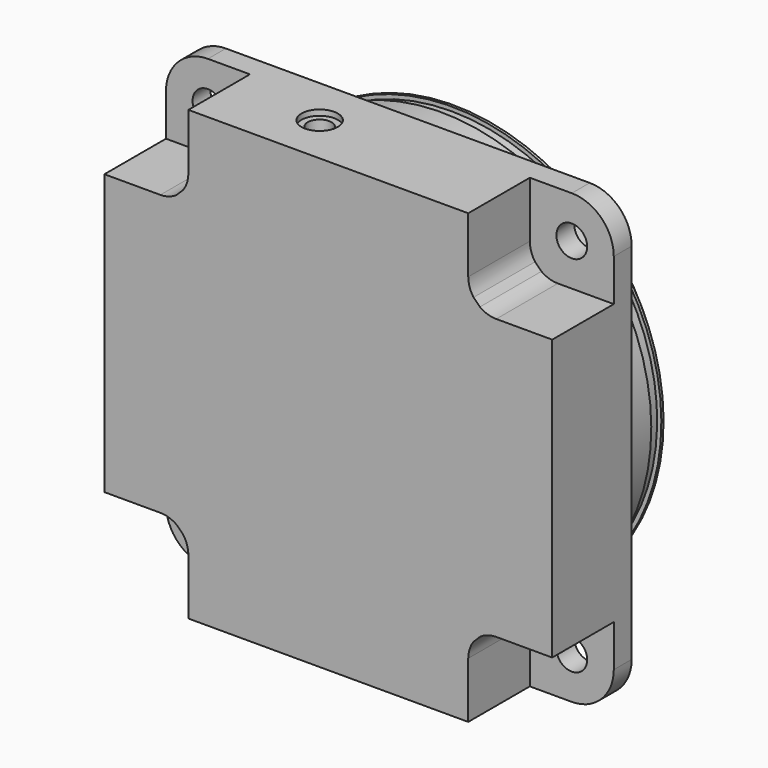
from build123d import *

# Parameters (mm, degrees)
F1_DEPTH        = 58
F0_R            = 5.5
F2_DEPTH        = 35.5
F3_DEPTH        = 35.5
F3_COPIES_COUNT = 4
F4_DEPTH        = 27.5
F4_COPIES_COUNT = 4
F5_SIZE         = 2
F7_D            = 8.5
F7_DEPTH        = 35
F7_CBORE_D      = 13
F7_CBORE_DEPTH  = 2
F7_TIP          = 2.5536576309
F9_D            = 8
F9_DEPTH        = 40
F9_TIP          = 2.4034424761
F10_W           = 4.5
F10_H           = 1.5


# Not quite as in the source:
# - a pattern or mirror of a feature is missing from the dataset's text; its kind, count and spacing are read off the source's solid


with BuildPart() as f1:
    # F0 (on Front) → F1 (new body)
    with BuildSketch(Plane.XZ):
        with BuildLine():
            ThreePointArc((-51.8845091547, 54.1571575119), (-52.9289321881, 52.9289321881), (-54.1571575119, 51.8845091547))
            ThreePointArc((-54.1571575119, 51.8845091547), (-27.9572279259, -69.5944926463), (75, 0))
            ThreePointArc((75, 0), (29.4419922338, 68.979483133), (-51.8845091547, 54.1571575119))
        make_face()
        with BuildLine():
            ThreePointArc((-51.8845091547, 54.1571575119), (-53.033008589, 53.033008589), (-54.1571575119, 51.8845091547))
            ThreePointArc((-54.1571575119, 51.8845091547), (-52.9289321881, 52.9289321881), (-51.8845091547, 54.1571575119))
        make_face()
    extrude(amount=-F1_DEPTH)

    # F0 (on Front) → F2 (join)
    with BuildSketch(Plane.XZ):
        with BuildLine():
            Line((-65, -80), (65, -80))
            ThreePointArc((65, -80), (75.6066017178, -75.6066017178), (80, -65))
            Line((80, -65), (80, 65))
            ThreePointArc((80, 65), (75.6066017178, 75.6066017178), (65, 80))
            Line((65, 80), (-50, 80))
            Line((-50, 80), (-50, 60))
            ThreePointArc((-50, 60), (-50.4827811717, 56.9303834484), (-51.8845091547, 54.1571575119))
            ThreePointArc((-51.8845091547, 54.1571575119), (29.4419922338, 68.979483133), (75, 0))
            ThreePointArc((75, 0), (-27.9572279259, -69.5944926463), (-54.1571575119, 51.8845091547))
            ThreePointArc((-54.1571575119, 51.8845091547), (-56.9303834484, 50.4827811717), (-60, 50))
            Line((-60, 50), (-80, 50))
            Line((-80, 50), (-80, -65))
            ThreePointArc((-80, -65), (-75.6066017178, -75.6066017178), (-65, -80))
        make_face()
        with BuildLine():
            Line((-80, 65), (-80, 50))
            Line((-80, 50), (-60, 50))
            ThreePointArc((-60, 50), (-56.9303834484, 50.4827811717), (-54.1571575119, 51.8845091547))
            ThreePointArc((-54.1571575119, 51.8845091547), (-53.033008589, 53.033008589), (-51.8845091547, 54.1571575119))
            ThreePointArc((-51.8845091547, 54.1571575119), (-50.4827811717, 56.9303834484), (-50, 60))
            Line((-50, 60), (-50, 80))
            Line((-50, 80), (-65, 80))
            ThreePointArc((-65, 80), (-75.6066017178, 75.6066017178), (-80, 65))
        make_face()
        with Locations((-65, 65)):
            Circle(F0_R, mode=Mode.SUBTRACT)
        with Locations((-65, 65)):
            Circle(F0_R)
    extrude(amount=-F2_DEPTH)

    # F0 (on Front) → F3 (cut, through all)
    with BuildSketch(Plane.XZ):
        with Locations((-65, 65)):
            Circle(F0_R)
    f3 = extrude(amount=-F3_DEPTH, mode=Mode.SUBTRACT)

    # F3_copies: F3 ×4 about axis
    f3_copies_axis = Axis((0, 0, 0), (0, 1, 0))
    for i in range(1, F3_COPIES_COUNT):
        add(f3.rotate(f3_copies_axis, i * 360 / F3_COPIES_COUNT), mode=Mode.SUBTRACT)

    # F0 (on Front) → F4 (cut)
    with BuildSketch(Plane.XZ):
        with BuildLine():
            Line((-80, 65), (-80, 50))
            Line((-80, 50), (-60, 50))
            ThreePointArc((-60, 50), (-56.9303834484, 50.4827811717), (-54.1571575119, 51.8845091547))
            ThreePointArc((-54.1571575119, 51.8845091547), (-53.033008589, 53.033008589), (-51.8845091547, 54.1571575119))
            ThreePointArc((-51.8845091547, 54.1571575119), (-50.4827811717, 56.9303834484), (-50, 60))
            Line((-50, 60), (-50, 80))
            Line((-50, 80), (-65, 80))
            ThreePointArc((-65, 80), (-75.6066017178, 75.6066017178), (-80, 65))
        make_face()
        with Locations((-65, 65)):
            Circle(F0_R, mode=Mode.SUBTRACT)
    f4 = extrude(amount=-F4_DEPTH, mode=Mode.SUBTRACT)

    # F4_copies: F4 ×4 about axis
    f4_copies_axis = Axis((0, 0, 0), (0, 1, 0))
    for i in range(1, F4_COPIES_COUNT):
        add(f4.rotate(f4_copies_axis, i * 360 / F4_COPIES_COUNT), mode=Mode.SUBTRACT)

    # F5
    f5_edges = [f1.edges().sort_by_distance(p)[0] for p in [
        (-75, 58, 0),
    ]]
    chamfer(f5_edges, length=F5_SIZE)

    # F7
    with Locations(Plane.XY.offset(80)):
        with Locations((-17.5, 18)):
            CounterBoreHole(F7_D / 2, F7_CBORE_D / 2, F7_CBORE_DEPTH, depth=F7_DEPTH)
            with Locations((0, 0, -(F7_DEPTH + F7_TIP / 2))):  # 118° drill point
                Cone(0, F7_D / 2, F7_TIP, mode=Mode.SUBTRACT)

    # F9
    with Locations(Plane(origin=(0, 58, 0), x_dir=(-1, 0, 0), z_dir=(0, 1, 0))):
        with Locations((17.5, 50)):
            Hole(F9_D / 2, depth=F9_DEPTH)
            with Locations((0, 0, -(F9_DEPTH + F9_TIP / 2))):  # 118° drill point
                Cone(0, F9_D / 2, F9_TIP, mode=Mode.SUBTRACT)

    # F10 (on Right) → F11 (revolve, cut)
    with BuildSketch(Plane.YZ):
        with Locations((52.75, 74.25)):
            Rectangle(F10_W, F10_H)
    revolve(axis=Axis((0, 29, 0), (0, 1, 0)), mode=Mode.SUBTRACT)


solid = f1.part
